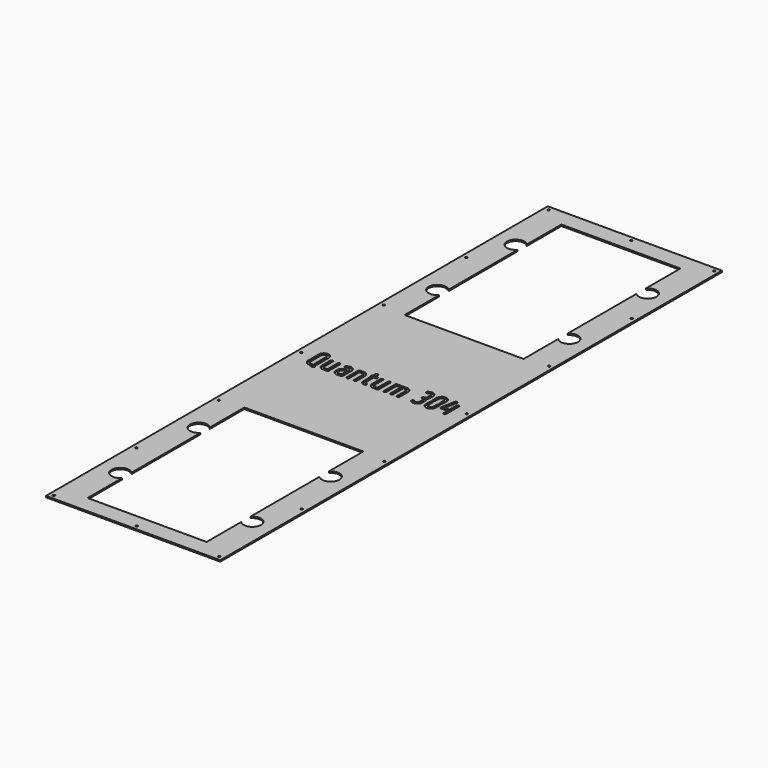
from build123d import *

# Parameters (mm, degrees)
F0_W     = 254
F0_H     = 914.4
F0_R     = 1.5750032
F1_DEPTH = 2.032


# Not quite as in the source:
# - ends of sketch curves that miss each other by under 0.0002 mm in the source are joined


with BuildPart() as f1:
    # F0 (on Top) → F1 (new body)
    with BuildSketch(Plane.XY):
        Rectangle(F0_W, F0_H)
        with Locations((-120.65, -450.85)):
            Circle(F0_R, mode=Mode.SUBTRACT)
        with Locations((-120.65, -300.5666582)):
            Circle(F0_R, mode=Mode.SUBTRACT)
        with Locations((-120.65, -150.2833418)):
            Circle(F0_R, mode=Mode.SUBTRACT)
        Polygon((-88.2005348, -19.8040498), (-88.2997472, -19.8288656), (-88.4237754, -19.853656), (-88.5229878, -19.8784718), (-88.6222002, -19.8784718), (-88.7214126, -19.8784718), (-88.7958346, -19.8784718), (-88.895047, -19.8784718), (-88.969469, -19.8784718), (-89.043891, -19.853656), (-89.1182876, -19.853656), (-89.1927096, -19.8288656), (-89.2671316, -19.8040498), (-89.366344, -19.7792594), (-97.1302096, -17.1251372), (-97.626297, -16.9515028), (-98.0727782, -16.753078), (-98.5192848, -16.5298374), (-98.9161598, -16.3065968), (-99.3130348, -16.0585404), (-99.685094, -15.810484), (-100.007547, -15.5376372), (-100.3300254, -15.24), (-100.8261128, -14.694281), (-101.272594, -14.1237716), (-101.6198628, -13.5284718), (-101.9423158, -12.9083562), (-102.1655564, -12.238609), (-102.3391908, -11.5688872), (-102.4384032, -10.8495592), (-102.463219, -10.1054154), (-102.463219, 9.2422472), (-102.4384032, 9.9615752), (-102.3391908, 10.6809032), (-102.1655564, 11.350625), (-101.9423158, 12.0203722), (-101.6198628, 12.6404878), (-101.272594, 13.2357876), (-100.8261128, 13.806297), (-100.3300254, 14.352016), (-99.7843064, 14.8481034), (-99.213797, 15.2945846), (-98.6184972, 15.6418534), (-97.9983816, 15.9643064), (-97.3286598, 16.187547), (-96.6589126, 16.3611814), (-95.9395846, 16.4603938), (-95.1954408, 16.4852096), (-94.4761128, 16.4603938), (-93.7567848, 16.3611814), (-93.0870376, 16.187547), (-92.4173158, 15.9643064), (-91.7972002, 15.6418534), (-91.2019004, 15.2945846), (-90.631391, 14.8481034), (-90.085672, 14.352016), (-89.5895846, 13.806297), (-89.1431034, 13.2357876), (-88.7958346, 12.6404878), (-88.4733816, 12.0203722), (-88.250141, 11.350625), (-88.0765066, 10.6809032), (-87.9772688, 9.9615752), (-87.9524784, 9.2422472), (-87.9524784, -10.1054154), (-87.9524784, -10.328656), (-87.9524784, -10.5518966), (-87.9772688, -10.7751372), (-88.0020846, -10.9983778), (-88.0269004, -11.196828), (-88.0516908, -11.4200686), (-88.0765066, -11.6184934), (-88.1261128, -11.841734), (-88.1509032, -11.9657622), (-88.2005348, -12.1146062), (-88.250141, -12.238609), (-88.2997472, -12.3626372), (-88.3741438, -12.461875), (-88.4485658, -12.5858778), (-88.5477782, -12.6851156), (-88.647016, -12.8091184), (-88.7958346, -12.9331466), (-88.969469, -13.0571748), (-89.1182876, -13.1563872), (-89.291922, -13.2308092), (-89.4655564, -13.3052312), (-89.6391908, -13.3548374), (-89.837641, -13.3796278), (-90.0360658, -13.3796278), (-90.234516, -13.3796278), (-90.4081504, -13.3548374), (-90.6065752, -13.3052312), (-90.7802096, -13.2308092), (-90.9290282, -13.1563872), (-91.1026626, -13.0571748), (-91.2515066, -12.9579624), (-91.4003252, -12.8091184), (-91.5243534, -12.6602998), (-91.6483816, -12.5114812), (-91.747594, -12.3626372), (-91.822016, -12.1890028), (-91.8964126, -12.0153684), (-91.9212284, -11.841734), (-91.9460188, -11.6433092), (-91.9708346, -11.444859), (-91.9708346, -11.3952528), (-91.9708346, -11.3456466), (-91.9708346, -11.2960404), (-91.9708346, -11.2464342), (-91.9460188, -11.196828), (-91.9460188, -11.122406), (-91.9460188, -11.0727998), (-91.9460188, -11.0231936), (-91.9212284, -10.8991654), (-91.8964126, -10.799953), (-91.8716222, -10.6759248), (-91.8468064, -10.5767124), (-91.8468064, -10.4526842), (-91.822016, -10.3534718), (-91.822016, -10.2294436), (-91.822016, -10.1054154), (-91.822016, 9.2422472), (-91.8468064, 9.5647002), (-91.8716222, 9.911969), (-91.9708346, 10.234422), (-92.070047, 10.5320846), (-92.218891, 10.8297472), (-92.3677096, 11.102594), (-92.5909502, 11.3754408), (-92.8141908, 11.6234972), (-93.0622472, 11.8467378), (-93.335094, 12.0699784), (-93.6079408, 12.218797), (-93.9056034, 12.367641), (-94.203266, 12.4668534), (-94.525719, 12.5660658), (-94.8729878, 12.5908816), (-95.1954408, 12.615672), (-95.5427096, 12.5908816), (-95.8899784, 12.5660658), (-96.2124314, 12.4668534), (-96.510094, 12.367641), (-96.8077566, 12.218797), (-97.0806034, 12.0699784), (-97.3534502, 11.8467378), (-97.6015066, 11.6234972), (-97.8247472, 11.3754408), (-98.0479878, 11.102594), (-98.1968064, 10.8297472), (-98.3456504, 10.5320846), (-98.4448628, 10.234422), (-98.5440752, 9.911969), (-98.568891, 9.5647002), (-98.5936814, 9.2422472), (-98.5936814, -10.1054154), (-98.568891, -10.4526842), (-98.5440752, -10.7751372), (-98.4696532, -11.0727998), (-98.3704408, -11.3704624), (-98.2216222, -11.6433092), (-98.0727782, -11.8913656), (-97.8743534, -12.1393966), (-97.6511128, -12.3626372), (-97.4278722, -12.5610874), (-97.1798158, -12.7595122), (-96.9317848, -12.9331466), (-96.6589126, -13.0819906), (-96.4108816, -13.2059934), (-96.113219, -13.3300216), (-95.8403722, -13.429234), (-95.5427096, -13.5284718), (-88.1261128, -16.1081466), (-87.9276626, -16.1825686), (-87.7540282, -16.281781), (-87.6052096, -16.3809934), (-87.456391, -16.5050216), (-87.307547, -16.6290498), (-87.1835188, -16.7778684), (-87.0843064, -16.9267124), (-86.985094, -17.1003468), (-86.9354878, -17.224375), (-86.910672, -17.3235874), (-86.8610658, -17.4227998), (-86.8362754, -17.546828), (-86.8114596, -17.6460404), (-86.8114596, -17.7452528), (-86.7866438, -17.8444906), (-86.7866438, -17.943703), (-86.7866438, -18.018125), (-86.7866438, -18.0925216), (-86.8114596, -18.1669436), (-86.8114596, -18.2413656), (-86.8362754, -18.3157622), (-86.8362754, -18.3901842), (-86.8610658, -18.4893966), (-86.8858816, -18.5638186), (-86.9602782, -18.737453), (-87.059516, -18.9110874), (-87.1587284, -19.0847218), (-87.2579408, -19.2335404), (-87.4067848, -19.3575686), (-87.5556034, -19.4815968), (-87.704422, -19.605625), (-87.8780564, -19.7048374), (-87.9772688, -19.7296278), (-88.101297, -19.7792594), align=None, mode=Mode.SUBTRACT)
        Polygon((-82.4954408, -11.0727998), (-82.5946532, -10.3782622), (-82.6442848, -9.6341184), (-82.6442848, 5.3727096), (-82.619469, 5.546344), (-82.5946532, 5.7447688), (-82.545047, 5.9184032), (-82.4954408, 6.0920376), (-82.4210188, 6.265672), (-82.3218064, 6.4393064), (-82.1977782, 6.588125), (-82.0737754, 6.736969), (-81.9249314, 6.8609972), (-81.7761128, 6.985), (-81.6024784, 7.0842378), (-81.428844, 7.1586344), (-81.2552096, 7.208266), (-81.0815752, 7.2578722), (-80.8831504, 7.2826626), (-80.709516, 7.3074784), (-80.5110658, 7.2826626), (-80.312641, 7.2578722), (-80.1390066, 7.208266), (-79.9653722, 7.1586344), (-79.7917378, 7.0842378), (-79.6181034, 6.985), (-79.4692848, 6.8609972), (-79.3204408, 6.736969), (-79.1964126, 6.588125), (-79.0724098, 6.4393064), (-78.973172, 6.265672), (-78.8987754, 6.0920376), (-78.8491438, 5.9184032), (-78.7995376, 5.7447688), (-78.7747472, 5.546344), (-78.7747472, 5.3727096), (-78.7747472, -9.6341184), (-78.7499314, -9.9813872), (-78.7003252, -10.3038656), (-78.6259032, -10.6263186), (-78.5266908, -10.9239812), (-78.3778722, -11.2216184), (-78.2042378, -11.4944906), (-78.0057876, -11.7673374), (-77.782547, -12.0401842), (-77.5097002, -12.2634248), (-77.2368534, -12.461875), (-76.9640066, -12.635484), (-76.666344, -12.784328), (-76.3686814, -12.8835404), (-76.0462284, -12.9579624), (-75.7237754, -13.0075686), (-75.3765066, -13.032359), (-71.978266, -13.032359), (-71.978266, 5.3727096), (-71.978266, 5.546344), (-71.9534502, 5.7447688), (-71.903844, 5.9184032), (-71.8542378, 6.0920376), (-71.7798158, 6.265672), (-71.6806034, 6.4393064), (-71.5565752, 6.588125), (-71.432547, 6.736969), (-71.2837284, 6.8609972), (-71.1349098, 6.985), (-70.9612754, 7.0842378), (-70.787641, 7.1586344), (-70.6140066, 7.208266), (-70.4403722, 7.2578722), (-70.241922, 7.2826626), (-70.0434972, 7.3074784), (-69.8698628, 7.2826626), (-69.6714126, 7.2578722), (-69.4977782, 7.208266), (-69.3241438, 7.1586344), (-69.1505348, 7.0842378), (-68.9769004, 6.985), (-68.8280564, 6.8609972), (-68.6792378, 6.736969), (-68.5552096, 6.588125), (-68.4311814, 6.4393064), (-68.331969, 6.265672), (-68.257547, 6.0920376), (-68.2079408, 5.9184032), (-68.1583346, 5.7447688), (-68.1335188, 5.546344), (-68.1087284, 5.3727096), (-68.1087284, -14.9671278), (-68.1335188, -15.1407622), (-68.1583346, -15.3392124), (-68.2079408, -15.5128468), (-68.257547, -15.6864812), (-68.331969, -15.8601156), (-68.4311814, -16.03375), (-68.5552096, -16.1825686), (-68.6792378, -16.3313872), (-68.8280564, -16.4554154), (-68.9769004, -16.5794436), (-69.1505348, -16.678656), (-69.3241438, -16.753078), (-69.4977782, -16.8026842), (-69.6714126, -16.8522904), (-69.8698628, -16.8771062), (-70.0434972, -16.9018966), (-75.3765066, -16.9018966), (-76.1206504, -16.8522904), (-76.8151626, -16.753078), (-77.5097002, -16.5794436), (-78.1546316, -16.356203), (-78.7747472, -16.0585404), (-79.3948628, -15.6864812), (-79.9653722, -15.2647904), (-80.5110658, -14.768703), (-81.0071532, -14.222984), (-81.428844, -13.6525), (-81.8009032, -13.032359), (-82.0985658, -12.4122434), (-82.3218064, -11.7673374), align=None, mode=Mode.SUBTRACT)
        Polygon((-62.304422, -7.6745592), (-62.2796316, -6.9304154), (-62.1803938, -6.2358778), (-62.0067848, -5.5413656), (-61.7835188, -4.8964342), (-61.4610658, -4.2763186), (-61.113797, -3.656203), (-60.6673158, -3.0856936), (-60.1712284, -2.54), (-59.6999314, -2.0934934), (-59.1790282, -1.7214342), (-58.6581504, -1.3741654), (-58.1124314, -1.0765028), (-57.541922, -0.8532622), (-56.9466222, -0.6548374), (-56.3265066, -0.5308092), (-55.706391, -0.4315968), (-55.4583346, -0.4563872), (-55.235094, -0.481203), (-55.0366438, -0.5308092), (-54.838219, -0.5804154), (-54.6397688, -0.6796278), (-54.4661598, -0.7788656), (-54.3173158, -0.878078), (-54.1684972, -1.0268966), (-54.044469, -1.1757406), (-53.9204408, -1.3245592), (-53.8212284, -1.4981936), (-53.7468064, -1.6470122), (-53.6724098, -1.8206466), (-53.6227782, -1.994281), (-53.5979878, -2.1927312), (-53.5979878, -2.3663656), (-53.5979878, -2.5647904), (-53.6227782, -2.7632406), (-53.6724098, -2.936875), (-53.7468064, -3.110484), (-53.8212284, -3.2841184), (-53.9204408, -3.4329624), (-54.0196532, -3.581781), (-54.1436814, -3.730625), (-54.2925254, -3.8546278), (-54.4165282, -3.9538656), (-54.5653722, -4.053078), (-54.7141908, -4.1275), (-54.8630348, -4.2018966), (-55.0118534, -4.2515028), (-55.160672, -4.2763186), (-55.3343064, -4.301109), (-55.631969, -4.3507406), (-55.9296316, -4.4003468), (-56.2024784, -4.4747434), (-56.4753252, -4.5987716), (-56.7233816, -4.7227998), (-56.9714126, -4.8964342), (-57.219469, -5.0700686), (-57.4427096, -5.2933092), (-57.6659502, -5.5413656), (-57.8891908, -5.8142124), (-58.0380348, -6.0870592), (-58.1868534, -6.3847218), (-58.2860658, -6.682359), (-58.3852782, -7.0048374), (-58.410094, -7.3272904), (-58.4349098, -7.6745592), (-58.4349098, -9.6341184), (-58.410094, -9.9813872), (-58.3852782, -10.3038656), (-58.2860658, -10.6263186), (-58.1868534, -10.9239812), (-58.0380348, -11.2216184), (-57.8891908, -11.4944906), (-57.6659502, -11.7673374), (-57.4427096, -12.0401842), (-57.1946532, -12.2634248), (-56.9218064, -12.461875), (-56.6489596, -12.635484), (-56.351297, -12.784328), (-56.0536598, -12.8835404), (-55.7311814, -12.9579624), (-55.3839126, -13.0075686), (-55.0366438, -13.032359), (-51.663219, -13.032359), (-51.663219, 0.5109972), (-51.6880348, 0.8334502), (-51.737641, 1.180719), (-51.8120376, 1.503172), (-51.9360658, 1.8008346), (-52.060094, 2.0984972), (-52.2337284, 2.371344), (-52.4321532, 2.6441908), (-52.6553938, 2.8922472), (-52.928266, 3.1154878), (-53.176297, 3.3387284), (-53.4739596, 3.487547), (-53.7468064, 3.636391), (-54.0692848, 3.7356034), (-54.3917378, 3.8348158), (-54.7141908, 3.8596316), (-55.0614596, 3.884422), (-55.4087284, 3.8596316), (-55.7559972, 3.81), (-56.0784502, 3.7356034), (-56.3761128, 3.636391), (-56.6737754, 3.487547), (-56.9714126, 3.3139126), (-57.2442848, 3.1154878), (-57.5171316, 2.8674314), (-57.6411598, 2.7434032), (-57.7899784, 2.619375), (-57.9636128, 2.5201626), (-58.1124314, 2.445766), (-58.2860658, 2.371344), (-58.484516, 2.3217378), (-58.6581504, 2.296922), (-58.881391, 2.296922), (-59.0550254, 2.296922), (-59.2534502, 2.3217378), (-59.4270846, 2.371344), (-59.600719, 2.4209502), (-59.7743534, 2.5201626), (-59.9479878, 2.619375), (-60.0968064, 2.7186128), (-60.2456504, 2.8674314), (-60.3696532, 2.9914596), (-60.4936814, 3.165094), (-60.5928938, 3.3139126), (-60.6673158, 3.487547), (-60.716922, 3.6611814), (-60.7665282, 3.8348158), (-60.791344, 4.033266), (-60.8161598, 4.2316908), (-60.791344, 4.4053252), (-60.7665282, 4.60375), (-60.716922, 4.7773844), (-60.6673158, 4.9510188), (-60.5928938, 5.1246532), (-60.4936814, 5.2734972), (-60.3696532, 5.4223158), (-60.2456504, 5.5711344), (-59.6999314, 6.0920376), (-59.1046316, 6.5385188), (-58.5093064, 6.9106034), (-57.8644004, 7.2330564), (-57.1946532, 7.4811128), (-56.5249314, 7.6299314), (-55.8056034, 7.7539596), (-55.0614596, 7.77875), (-54.3421316, 7.7539596), (-53.6227782, 7.6547472), (-52.9530564, 7.4811128), (-52.2833346, 7.2578722), (-51.663219, 6.9353938), (-51.0678938, 6.588125), (-50.4974098, 6.1416438), (-49.9516908, 5.6455564), (-49.4556034, 5.0998628), (-49.0091222, 4.5293534), (-48.6370376, 3.9340282), (-48.3394004, 3.2891222), (-48.1161598, 2.6441908), (-47.9425254, 1.9496532), (-47.8432876, 1.2303252), (-47.7936814, 0.5109972), (-47.7936814, -14.9671278), (-47.7936814, -15.1407622), (-47.8184972, -15.3392124), (-47.8681034, -15.5128468), (-47.9425254, -15.6864812), (-48.016922, -15.8601156), (-48.1161598, -16.03375), (-48.2401626, -16.1825686), (-48.3641908, -16.3313872), (-48.5130348, -16.4554154), (-48.6618534, -16.5794436), (-48.810672, -16.678656), (-48.9843064, -16.753078), (-49.1579408, -16.8026842), (-49.3315752, -16.8522904), (-49.5300254, -16.8771062), (-49.7284502, -16.9018966), (-55.0366438, -16.9018966), (-55.7807876, -16.8522904), (-56.500141, -16.753078), (-57.1698628, -16.5794436), (-57.8395846, -16.356203), (-58.4597002, -16.0585404), (-59.0550254, -15.6864812), (-59.6255348, -15.2647904), (-60.1712284, -14.768703), (-60.6673158, -14.222984), (-61.113797, -13.6525), (-61.4610658, -13.032359), (-61.7835188, -12.4122434), (-62.0067848, -11.7673374), (-62.1803938, -11.0727998), (-62.2796316, -10.3782622), (-62.304422, -9.6341184), align=None, mode=Mode.SUBTRACT)
        Polygon((-42.3862754, 5.9184032), (-42.3118534, 6.0920376), (-42.2374314, 6.265672), (-42.138219, 6.4393064), (-42.0141908, 6.588125), (-41.8901626, 6.736969), (-41.741344, 6.8609972), (-41.5925254, 6.985), (-41.4436814, 7.0842378), (-41.270047, 7.1586344), (-41.0964126, 7.208266), (-40.9227782, 7.2578722), (-40.7243534, 7.2826626), (-40.5259032, 7.3074784), (-35.2177096, 7.3074784), (-34.4735658, 7.2578722), (-33.7542378, 7.1586344), (-33.084516, 6.985), (-32.4147688, 6.7617594), (-31.7946532, 6.4641222), (-31.1993534, 6.0920376), (-30.628844, 5.6703722), (-30.0831504, 5.1742594), (-29.5870376, 4.6285658), (-29.1405564, 4.0580564), (-28.7932876, 3.4379408), (-28.4708346, 2.8178252), (-28.247594, 2.1728938), (-28.0739596, 1.4783816), (-27.9747472, 0.783844), (-27.9499314, 0.0397002), (-27.9499314, -14.9671278), (-27.9499314, -15.1407622), (-27.9747472, -15.3392124), (-28.0243534, -15.5128468), (-28.0987754, -15.6864812), (-28.173172, -15.8601156), (-28.2724098, -16.03375), (-28.3964126, -16.1825686), (-28.5204408, -16.3313872), (-28.6692848, -16.4554154), (-28.8181034, -16.5794436), (-28.966922, -16.678656), (-29.1405564, -16.753078), (-29.3141908, -16.8026842), (-29.4878252, -16.8522904), (-29.6862754, -16.8771062), (-29.8847002, -16.9018966), (-30.0831504, -16.8771062), (-30.2815752, -16.8522904), (-30.4552096, -16.8026842), (-30.628844, -16.753078), (-30.8024784, -16.678656), (-30.951297, -16.5794436), (-31.100141, -16.4554154), (-31.2489596, -16.3313872), (-31.3729878, -16.1825686), (-31.497016, -16.03375), (-31.5962284, -15.8601156), (-31.6706504, -15.6864812), (-31.745047, -15.5128468), (-31.7946532, -15.3392124), (-31.819469, -15.1407622), (-31.819469, -14.9671278), (-31.819469, 0.0397002), (-31.8442848, 0.386969), (-31.8690752, 0.709422), (-31.9682876, 1.031875), (-32.0675254, 1.3295376), (-32.216344, 1.6272002), (-32.3651626, 1.900047), (-32.5884032, 2.1728938), (-32.8116438, 2.445766), (-33.0597002, 2.6690066), (-33.332547, 2.8674314), (-33.6053938, 3.0410658), (-33.9030564, 3.1898844), (-34.200719, 3.2891222), (-34.523172, 3.3635188), (-34.8704408, 3.413125), (-35.2177096, 3.4379408), (-38.5911598, 3.4379408), (-38.5911598, -14.9671278), (-38.5911598, -15.1407622), (-38.6159502, -15.3392124), (-38.6655564, -15.5128468), (-38.7399784, -15.6864812), (-38.8144004, -15.8601156), (-38.9136128, -16.03375), (-39.037641, -16.1825686), (-39.1616438, -16.3313872), (-39.3104878, -16.4554154), (-39.4593064, -16.5794436), (-39.6081504, -16.678656), (-39.7817848, -16.753078), (-39.9553938, -16.8026842), (-40.1290282, -16.8522904), (-40.3274784, -16.8771062), (-40.5259032, -16.9018966), (-40.7243534, -16.8771062), (-40.9227782, -16.8522904), (-41.0964126, -16.8026842), (-41.270047, -16.753078), (-41.4436814, -16.678656), (-41.5925254, -16.5794436), (-41.741344, -16.4554154), (-41.8901626, -16.3313872), (-42.0141908, -16.1825686), (-42.138219, -16.03375), (-42.2374314, -15.8601156), (-42.3118534, -15.6864812), (-42.3862754, -15.5128468), (-42.4358816, -15.3392124), (-42.460672, -15.1407622), (-42.460672, -14.9671278), (-42.460672, 5.3727096), (-42.460672, 5.546344), (-42.4358816, 5.7447688), align=None, mode=Mode.SUBTRACT)
        Polygon((-22.3440752, 3.81), (-22.4432876, 3.9092378), (-22.5425254, 4.0084502), (-22.691344, 4.1572688), (-22.7905564, 4.3061128), (-22.8897688, 4.4797472), (-22.9890066, 4.6285658), (-23.0386128, 4.8022002), (-23.088219, 4.9758346), (-23.1130348, 5.1742594), (-23.1130348, 5.3727096), (-23.1130348, 5.546344), (-23.088219, 5.7447688), (-23.0386128, 5.9184032), (-22.9890066, 6.0920376), (-22.8897688, 6.265672), (-22.7905564, 6.4393064), (-22.691344, 6.588125), (-22.5425254, 6.736969), (-22.4432876, 6.8361814), (-22.3440752, 6.9106034), (-22.2448628, 6.985), (-22.1208346, 7.059422), (-22.0216222, 7.1090282), (-21.897594, 7.1586344), (-21.7735658, 7.208266), (-21.6495376, 7.2578722), (-21.6495376, 11.1522002), (-21.6495376, 11.3258346), (-21.6247472, 11.5242594), (-21.575141, 11.6978938), (-21.500719, 11.8715282), (-21.426297, 12.0451626), (-21.3270846, 12.218797), (-21.2030564, 12.367641), (-21.0790282, 12.5164596), (-20.9302096, 12.6404878), (-20.7565752, 12.764516), (-20.6077566, 12.8637284), (-20.4341222, 12.938125), (-20.2604878, 12.9877566), (-20.0868534, 13.0373628), (-19.913219, 13.0621532), (-19.7147688, 13.086969), (-19.516344, 13.0621532), (-19.3178938, 13.0373628), (-19.1442848, 12.9877566), (-18.9706504, 12.938125), (-18.797016, 12.8637284), (-18.648172, 12.764516), (-18.4993534, 12.6404878), (-18.3505348, 12.5164596), (-18.2265066, 12.367641), (-18.1024784, 12.218797), (-18.003266, 12.0451626), (-17.928844, 11.8715282), (-17.854422, 11.6978938), (-17.8048158, 11.5242594), (-17.7800254, 11.3258346), (-17.7800254, 11.1522002), (-17.7800254, 7.3074784), (-15.3491438, 7.3074784), (-15.1755348, 7.2826626), (-14.9770846, 7.2578722), (-14.8034502, 7.208266), (-14.6298158, 7.1586344), (-14.4561814, 7.0842378), (-14.282547, 6.985), (-14.1337284, 6.8609972), (-13.9849098, 6.736969), (-13.8608816, 6.588125), (-13.7368534, 6.4393064), (-13.637641, 6.265672), (-13.563219, 6.0920376), (-13.5136128, 5.9184032), (-13.4640066, 5.7447688), (-13.4391908, 5.546344), (-13.4144004, 5.3727096), (-13.4391908, 5.1742594), (-13.4640066, 4.9758346), (-13.5136128, 4.8022002), (-13.563219, 4.6285658), (-13.637641, 4.4549314), (-13.7368534, 4.281297), (-13.8608816, 4.1324784), (-13.9849098, 3.9836344), (-14.1337284, 3.8596316), (-14.282547, 3.7356034), (-14.4561814, 3.636391), (-14.6298158, 3.561969), (-14.8034502, 3.5123628), (-14.9770846, 3.4627566), (-15.1755348, 3.4379408), (-15.3491438, 3.4379408), (-17.7800254, 3.4379408), (-17.7800254, -10.6015028), (-17.7800254, -10.8495592), (-17.7303938, -11.0976156), (-17.6807876, -11.3208562), (-17.606391, -11.5440968), (-17.5071532, -11.7425216), (-17.3831504, -11.9409718), (-17.2343064, -12.1393966), (-17.0854878, -12.313031), (-16.8870376, -12.4866654), (-16.7134032, -12.635484), (-16.5149784, -12.7347218), (-16.2917378, -12.8339342), (-16.0684972, -12.9331466), (-15.8452566, -12.9827528), (-15.622016, -13.0075686), (-15.3491438, -13.032359), (-15.150719, -13.032359), (-14.9770846, -13.0571748), (-14.7786598, -13.106781), (-14.6050254, -13.1563872), (-14.431391, -13.255625), (-14.282547, -13.3548374), (-14.1089126, -13.4540498), (-13.960094, -13.6028684), (-13.8360658, -13.7517124), (-13.7120376, -13.900531), (-13.6128252, -14.0741654), (-13.5384032, -14.222984), (-13.488797, -14.3966184), (-13.4391908, -14.5702528), (-13.4144004, -14.768703), (-13.4144004, -14.9671278), (-13.4144004, -15.1407622), (-13.4391908, -15.3392124), (-13.488797, -15.5128468), (-13.5384032, -15.6864812), (-13.6128252, -15.8601156), (-13.7120376, -16.03375), (-13.8360658, -16.1825686), (-13.960094, -16.3313872), (-14.1089126, -16.4554154), (-14.282547, -16.5794436), (-14.431391, -16.678656), (-14.6050254, -16.753078), (-14.7786598, -16.8026842), (-14.9770846, -16.8522904), (-15.150719, -16.8771062), (-15.3491438, -16.9018966), (-15.9940752, -16.8522904), (-16.6141908, -16.7778684), (-17.209516, -16.6290498), (-17.7552096, -16.430625), (-18.3009032, -16.1577528), (-18.8218064, -15.8601156), (-19.3178938, -15.4632406), (-19.7891908, -15.0415498), (-20.235672, -14.5702528), (-20.6077566, -14.0741654), (-20.9302096, -13.5532622), (-21.178266, -13.0075686), (-21.4015066, -12.4370592), (-21.5255348, -11.841734), (-21.6247472, -11.2464342), (-21.6495376, -10.6015028), (-21.6495376, 3.4627566), (-21.7735658, 3.5123628), (-21.897594, 3.561969), (-22.0216222, 3.6115752), (-22.1208346, 3.6611814), (-22.2448628, 3.7356034), align=None, mode=Mode.SUBTRACT)
        Polygon((-9.4208346, -11.0727998), (-9.520047, -10.3782622), (-9.5696532, -9.6341184), (-9.5696532, 5.3727096), (-9.5448628, 5.546344), (-9.520047, 5.7447688), (-9.4704408, 5.9184032), (-9.4208346, 6.0920376), (-9.3464126, 6.265672), (-9.2472002, 6.4393064), (-9.123172, 6.588125), (-8.9991438, 6.736969), (-8.8503252, 6.8609972), (-8.7015066, 6.985), (-8.5278722, 7.0842378), (-8.3542378, 7.1586344), (-8.1806034, 7.208266), (-8.006969, 7.2578722), (-7.8085188, 7.2826626), (-7.6349098, 7.3074784), (-7.4364596, 7.2826626), (-7.2380348, 7.2578722), (-7.0644004, 7.208266), (-6.890766, 7.1586344), (-6.7171316, 7.0842378), (-6.5434972, 6.985), (-6.3946532, 6.8609972), (-6.2458346, 6.736969), (-6.1218064, 6.588125), (-5.9977782, 6.4393064), (-5.8985658, 6.265672), (-5.8241438, 6.0920376), (-5.7745376, 5.9184032), (-5.7249314, 5.7447688), (-5.700141, 5.546344), (-5.700141, 5.3727096), (-5.700141, -9.6341184), (-5.6753252, -9.9813872), (-5.625719, -10.3038656), (-5.551297, -10.6263186), (-5.4520846, -10.9239812), (-5.303266, -11.2216184), (-5.1296316, -11.4944906), (-4.9311814, -11.7673374), (-4.7079408, -12.0401842), (-4.435094, -12.2634248), (-4.1622472, -12.461875), (-3.8894004, -12.635484), (-3.5917378, -12.784328), (-3.2940752, -12.8835404), (-2.9716222, -12.9579624), (-2.6491438, -13.0075686), (-2.3019004, -13.032359), (1.0963402, -13.032359), (1.0963402, 5.3727096), (1.0963402, 5.546344), (1.121156, 5.7447688), (1.1707622, 5.9184032), (1.2203684, 6.0920376), (1.2947904, 6.265672), (1.3940028, 6.4393064), (1.518031, 6.588125), (1.6420592, 6.736969), (1.7908778, 6.8609972), (1.9397218, 6.985), (2.1133562, 7.0842378), (2.2869652, 7.1586344), (2.4605996, 7.208266), (2.634234, 7.2578722), (2.8326842, 7.2826626), (3.031109, 7.3074784), (3.2047434, 7.2826626), (3.4031936, 7.2578722), (3.576828, 7.208266), (3.7504624, 7.1586344), (3.9240968, 7.0842378), (4.0977312, 6.985), (4.2465498, 6.8609972), (4.3953684, 6.736969), (4.5193966, 6.588125), (4.6434248, 6.4393064), (4.7426372, 6.265672), (4.8170592, 6.0920376), (4.8666654, 5.9184032), (4.9162716, 5.7447688), (4.9410874, 5.546344), (4.9658778, 5.3727096), (4.9658778, -14.9671278), (4.9410874, -15.1407622), (4.9162716, -15.3392124), (4.8666654, -15.5128468), (4.8170592, -15.6864812), (4.7426372, -15.8601156), (4.6434248, -16.03375), (4.5193966, -16.1825686), (4.3953684, -16.3313872), (4.2465498, -16.4554154), (4.0977312, -16.5794436), (3.9240968, -16.678656), (3.7504624, -16.753078), (3.576828, -16.8026842), (3.4031936, -16.8522904), (3.2047434, -16.8771062), (3.031109, -16.9018966), (-2.3019004, -16.9018966), (-3.0460188, -16.8522904), (-3.7405564, -16.753078), (-4.435094, -16.5794436), (-5.0800254, -16.356203), (-5.700141, -16.0585404), (-6.3202566, -15.6864812), (-6.890766, -15.2647904), (-7.4364596, -14.768703), (-7.932547, -14.222984), (-8.3542378, -13.6525), (-8.726297, -13.032359), (-9.0239596, -12.4122434), (-9.2472002, -11.7673374), align=None, mode=Mode.SUBTRACT)
        with Locations((0, -450.85)):
            Circle(F0_R, mode=Mode.SUBTRACT)
        with BuildLine():
            Line((-86.7791, -209.0872374), (-86.7791, -146.05))
            Line((-86.7791, -146.05), (86.7791, -146.05))
            Line((86.7791, -146.05), (86.7791, -209.0872374))
            ThreePointArc((86.7791, -209.0872374), (109.0041, -217.4875), (86.7791010851, -225.887761643))
            Line((86.7791010851, -225.887761643), (86.7791, -351.9622374))
            ThreePointArc((86.7791, -351.9622374), (109.0041, -360.3625), (86.7791010851, -368.762761643))
            Line((86.7791010851, -368.762761643), (86.7791, -431.8))
            Line((86.7791, -431.8), (-86.7791, -431.8))
            Line((-86.7791, -431.8), (-86.7791, -368.7627626))
            ThreePointArc((-86.7791, -368.7627626), (-109.0041, -360.3625), (-86.7791010851, -351.962238357))
            Line((-86.7791010851, -351.962238357), (-86.7791, -225.8877626))
            ThreePointArc((-86.7791, -225.8877626), (-109.0041, -217.4875), (-86.7791, -209.0872374))
        make_face(mode=Mode.SUBTRACT)
        with Locations((120.65, -450.85)):
            Circle(F0_R, mode=Mode.SUBTRACT)
        with Locations((120.65, -300.5666582)):
            Circle(F0_R, mode=Mode.SUBTRACT)
        Polygon((11.8863872, -15.6864812), (11.8119652, -15.5128468), (11.762359, -15.3392124), (11.7375686, -15.1407622), (11.7375686, -14.9671278), (11.7375686, 5.3727096), (11.7375686, 5.546344), (11.762359, 5.7447688), (11.8119652, 5.9184032), (11.8863872, 6.0920376), (11.9608092, 6.265672), (12.0600216, 6.4393064), (12.1840498, 6.588125), (12.308078, 6.736969), (12.4568966, 6.8609972), (12.6057152, 6.985), (12.7545592, 7.0842378), (12.9281936, 7.1586344), (13.101828, 7.208266), (13.2754624, 7.2578722), (13.4738872, 7.2826626), (13.6723374, 7.3074784), (27.711781, 7.3074784), (28.431109, 7.2578722), (29.1504624, 7.1586344), (29.8201842, 6.985), (30.489906, 6.7617594), (31.1100216, 6.4641222), (31.7053468, 6.0920376), (32.2758562, 5.6703722), (32.8215498, 5.1742594), (33.3176372, 4.6285658), (33.7641184, 4.0580564), (34.1113872, 3.4379408), (34.4338402, 2.8178252), (34.6571062, 2.1728938), (34.8307152, 1.4783816), (34.929953, 0.783844), (34.9547434, 0.0397002), (34.9547434, -14.9671278), (34.9547434, -15.1407622), (34.929953, -15.3392124), (34.8803468, -15.5128468), (34.8059248, -15.6864812), (34.7315028, -15.8601156), (34.6322904, -16.03375), (34.5082622, -16.1825686), (34.384234, -16.3313872), (34.2354154, -16.4554154), (34.0865968, -16.5794436), (33.9377528, -16.678656), (33.7641184, -16.753078), (33.590484, -16.8026842), (33.4168496, -16.8522904), (33.2184248, -16.8771062), (33.0199746, -16.9018966), (32.8215498, -16.8771062), (32.6230996, -16.8522904), (32.4494652, -16.8026842), (32.2758562, -16.753078), (32.1022218, -16.678656), (31.9533778, -16.5794436), (31.8045592, -16.4554154), (31.6557152, -16.3313872), (31.5317124, -16.1825686), (31.4076842, -16.03375), (31.3084718, -15.8601156), (31.2340498, -15.6864812), (31.1596278, -15.5128468), (31.1100216, -15.3392124), (31.0852312, -15.1407622), (31.0852312, -14.9671278), (31.0852312, 0.0397002), (31.0604154, 0.386969), (31.0355996, 0.709422), (30.9363872, 1.031875), (30.8371748, 1.3295376), (30.6883562, 1.6272002), (30.5395122, 1.900047), (30.3162716, 2.1728938), (30.093031, 2.445766), (29.8449746, 2.6690066), (29.5721278, 2.8674314), (29.299281, 3.0410658), (29.0016184, 3.1898844), (28.7039812, 3.2891222), (28.3815028, 3.3635188), (28.034234, 3.413125), (27.711781, 3.4379408), (25.2809248, 3.4379408), (25.2809248, -14.9671278), (25.2809248, -15.1407622), (25.256109, -15.3392124), (25.2065028, -15.5128468), (25.1321062, -15.6864812), (25.0576842, -15.8601156), (24.9584718, -16.03375), (24.8344436, -16.1825686), (24.7104154, -16.3313872), (24.5615968, -16.4554154), (24.4127528, -16.5794436), (24.2639342, -16.678656), (24.0902998, -16.753078), (23.9166654, -16.8026842), (23.743031, -16.8522904), (23.5446062, -16.8771062), (23.346156, -16.9018966), (23.1477312, -16.8771062), (22.949281, -16.8522904), (22.7756466, -16.8026842), (22.6020122, -16.753078), (22.4283778, -16.678656), (22.2795592, -16.5794436), (22.1307152, -16.4554154), (21.9818966, -16.3313872), (21.8578684, -16.1825686), (21.7338402, -16.03375), (21.6346278, -15.8601156), (21.5602312, -15.6864812), (21.4858092, -15.5128468), (21.436203, -15.3392124), (21.4113872, -15.1407622), (21.4113872, -14.9671278), (21.4113872, 3.4379408), (15.6071062, 3.4379408), (15.6071062, -14.9671278), (15.6071062, -15.1407622), (15.5822904, -15.3392124), (15.5326842, -15.5128468), (15.4582622, -15.6864812), (15.3838402, -15.8601156), (15.2846278, -16.03375), (15.1605996, -16.1825686), (15.0365968, -16.3313872), (14.8877528, -16.4554154), (14.7389342, -16.5794436), (14.5900902, -16.678656), (14.4164812, -16.753078), (14.2428468, -16.8026842), (14.0692124, -16.8522904), (13.8707622, -16.8771062), (13.6723374, -16.9018966), (13.4738872, -16.8771062), (13.2754624, -16.8522904), (13.101828, -16.8026842), (12.9281936, -16.753078), (12.7545592, -16.678656), (12.6057152, -16.5794436), (12.4568966, -16.4554154), (12.308078, -16.3313872), (12.1840498, -16.1825686), (12.0600216, -16.03375), (11.9608092, -15.8601156), align=None, mode=Mode.SUBTRACT)
        Polygon((51.052984, -14.3470122), (51.0033778, -14.1733778), (50.9785874, -13.974953), (50.9537716, -13.8013186), (50.9785874, -13.6028684), (51.0033778, -13.4044436), (51.052984, -13.2308092), (51.1025902, -13.0571748), (51.1770122, -12.8835404), (51.2762246, -12.7347218), (51.4002528, -12.5610874), (51.524281, -12.4370592), (51.6730996, -12.2882406), (51.8219436, -12.1890028), (51.995578, -12.0897904), (52.1692124, -11.990578), (52.3428468, -11.9409718), (52.5164812, -11.8913656), (52.714906, -11.8665498), (52.8885404, -11.8665498), (53.0869652, -11.8665498), (53.2854154, -11.8913656), (53.4590498, -11.9409718), (53.6326842, -11.990578), (53.8063186, -12.065), (53.979953, -12.1642124), (54.1287716, -12.2882406), (54.2775902, -12.4122434), (54.5504624, -12.6602998), (54.8233092, -12.8835404), (55.1209718, -13.0571748), (55.418609, -13.2059934), (55.7410874, -13.3300216), (56.0635404, -13.4044436), (56.4108092, -13.4540498), (56.7332622, -13.4788656), (57.1053468, -13.4540498), (57.4277998, -13.429234), (57.7502528, -13.3300216), (58.0479154, -13.2308092), (58.345578, -13.0819906), (58.6432152, -12.9331466), (58.8912716, -12.709906), (59.139328, -12.4866654), (59.387359, -12.238609), (59.5858092, -11.9657622), (59.7594436, -11.6929154), (59.8834718, -11.3952528), (59.9826842, -11.0976156), (60.0818966, -10.7751372), (60.1067124, -10.4526842), (60.1315028, -10.1054154), (60.1315028, -4.772406), (60.1315028, -4.524375), (60.0818966, -4.2763186), (60.0322904, -4.053078), (59.9578684, -3.8298374), (59.858656, -3.6313872), (59.7346278, -3.4329624), (59.6105996, -3.2345122), (59.4369652, -3.0608778), (59.2633562, -2.8872434), (59.064906, -2.7384248), (58.8664812, -2.6392124), (58.668031, -2.54), (58.4447904, -2.465578), (58.2215498, -2.391156), (57.9734934, -2.3663656), (57.7254624, -2.3663656), (57.7006466, -2.3663656), (57.5270122, -2.3415498), (57.3285874, -2.316734), (57.154953, -2.2671278), (56.9813186, -2.2175216), (56.8076842, -2.1183092), (56.6340498, -2.0190968), (56.4852312, -1.919859), (56.3363872, -1.7710404), (56.212359, -1.6222218), (56.0883562, -1.4733778), (55.9891184, -1.2997434), (55.9147218, -1.1509248), (55.8650902, -0.9772904), (55.815484, -0.803656), (55.7906936, -0.6052312), (55.7658778, -0.4315968), (55.7906936, -0.2331466), (55.815484, -0.0347218), (55.8650902, 0.1389126), (55.9147218, 0.312547), (55.9891184, 0.4861814), (56.0883562, 0.6598158), (56.212359, 0.8086344), (56.3363872, 0.9574784), (56.4852312, 1.0815066), (56.6340498, 1.2055094), (56.8076842, 1.3047472), (56.9813186, 1.3791438), (57.154953, 1.42875), (57.3285874, 1.4783816), (57.5270122, 1.503172), (57.7006466, 1.503172), (57.7254624, 1.503172), (57.9734934, 1.5279878), (58.2215498, 1.5527782), (58.4447904, 1.6023844), (58.668031, 1.7016222), (58.8664812, 1.8008346), (59.064906, 1.900047), (59.2633562, 2.048891), (59.4369652, 2.2225), (59.6105996, 2.3961344), (59.7346278, 2.5945846), (59.858656, 2.7930094), (59.9578684, 2.9914596), (60.0322904, 3.2147002), (60.0818966, 3.4379408), (60.1315028, 3.6859972), (60.1315028, 3.9340282), (60.1315028, 9.2422472), (60.1067124, 9.589516), (60.0818966, 9.911969), (59.9826842, 10.234422), (59.8834718, 10.5320846), (59.7594436, 10.8297472), (59.5858092, 11.102594), (59.387359, 11.3754408), (59.139328, 11.6234972), (58.8912716, 11.8467378), (58.6432152, 12.0699784), (58.345578, 12.218797), (58.0479154, 12.367641), (57.7502528, 12.4668534), (57.4277998, 12.5660658), (57.1053468, 12.5908816), (56.7332622, 12.615672), (56.4108092, 12.5908816), (56.0635404, 12.54125), (55.7410874, 12.4668534), (55.4434248, 12.367641), (55.1457622, 12.218797), (54.8480996, 12.0203722), (54.5504624, 11.821922), (54.2775902, 11.573891), (54.1287716, 11.4498628), (53.979953, 11.3258346), (53.8063186, 11.2266222), (53.6326842, 11.1522002), (53.4590498, 11.0777782), (53.2854154, 11.028172), (53.0869652, 11.0033816), (52.8885404, 11.0033816), (52.714906, 11.0033816), (52.5164812, 11.028172), (52.3428468, 11.0777782), (52.1692124, 11.1273844), (51.995578, 11.2266222), (51.8219436, 11.3258346), (51.6730996, 11.425047), (51.524281, 11.573891), (51.4002528, 11.6978938), (51.2762246, 11.8715282), (51.1770122, 12.0203722), (51.1025902, 12.1940066), (51.052984, 12.367641), (51.0033778, 12.54125), (50.9785874, 12.7397002), (50.9537716, 12.938125), (50.9785874, 13.1117594), (51.0033778, 13.3102096), (51.052984, 13.483844), (51.1025902, 13.6574784), (51.201828, 13.8311128), (51.3010404, 13.9799314), (51.4002528, 14.12875), (51.5490968, 14.277594), (52.1196062, 14.7984972), (52.6900902, 15.2697688), (53.3102312, 15.6418534), (53.9551372, 15.9643064), (54.6000686, 16.187547), (55.2946062, 16.3611814), (56.0139342, 16.4852096), (56.7332622, 16.51), (57.477406, 16.4852096), (58.196734, 16.3859972), (58.8664812, 16.2123628), (59.536203, 15.9891222), (60.1563186, 15.6666438), (60.7516184, 15.319375), (61.3221278, 14.8728938), (61.8678468, 14.3768064), (62.3639342, 13.8311128), (62.8104154, 13.2606034), (63.1576842, 12.6652782), (63.4801372, 12.0451626), (63.7033778, 11.3754408), (63.8770122, 10.705719), (63.9762246, 9.986391), (64.0010404, 9.2422472), (64.0010404, 3.9340282), (63.9762246, 3.2891222), (63.901828, 2.693797), (63.752984, 2.0984972), (63.5545592, 1.5527782), (63.3065028, 1.031875), (63.0088402, 0.5109972), (62.636781, 0.0397002), (62.239906, -0.4315968), (62.636781, -0.878078), (63.0088402, -1.349375), (63.3065028, -1.8702528), (63.5545592, -2.391156), (63.752984, -2.936875), (63.901828, -3.5321748), (63.9762246, -4.1275), (64.0010404, -4.772406), (64.0010404, -10.1054154), (63.9762246, -10.8495592), (63.8770122, -11.5688872), (63.7033778, -12.238609), (63.4801372, -12.9083562), (63.1576842, -13.5284718), (62.8104154, -14.1237716), (62.3639342, -14.694281), (61.8678468, -15.24), (61.3221278, -15.7360874), (60.7516184, -16.1825686), (60.1563186, -16.5298374), (59.536203, -16.8522904), (58.8664812, -17.075531), (58.196734, -17.2491654), (57.477406, -17.3483778), (56.7332622, -17.3731936), (56.0139342, -17.3483778), (55.2946062, -17.224375), (54.6000686, -17.0507406), (53.9551372, -16.8275), (53.3102312, -16.5050216), (52.6900902, -16.1329624), (52.1196062, -15.6616654), (51.5490968, -15.1407622), (51.4002528, -14.9919436), (51.3010404, -14.843125), (51.201828, -14.694281), (51.1025902, -14.5206466), align=None, mode=Mode.SUBTRACT)
        with Locations((120.65, -150.2833418)):
            Circle(F0_R, mode=Mode.SUBTRACT)
        Polygon((73.1787716, -10.4526842), (73.2283778, -10.799953), (73.3027998, -11.122406), (73.4020122, -11.4200686), (73.5508562, -11.7177312), (73.7244652, -11.990578), (73.9229154, -12.2634248), (74.146156, -12.5114812), (74.4190028, -12.7347218), (74.6918496, -12.9579624), (74.9647218, -13.106781), (75.262359, -13.255625), (75.5600216, -13.3548374), (75.8824746, -13.4540498), (76.204953, -13.4788656), (76.5522218, -13.503656), (76.8994652, -13.4788656), (77.2219436, -13.4540498), (77.5443966, -13.3548374), (77.8420592, -13.255625), (78.1397218, -13.106781), (78.4125686, -12.9579624), (78.6854154, -12.7347218), (78.9582622, -12.5114812), (79.1815028, -12.2634248), (79.379953, -11.990578), (79.5535874, -11.7177312), (79.702406, -11.4200686), (79.8016184, -11.122406), (79.8760404, -10.799953), (79.9256466, -10.4526842), (79.9504624, -10.1054154), (79.9504624, -3.3585404), (79.9504624, -3.184906), (79.9752528, -2.9864812), (80.024859, -2.8128468), (80.0744652, -2.6392124), (80.1488872, -2.465578), (80.2480996, -2.2919436), (80.3721278, -2.143125), (80.496156, -1.994281), (80.6449746, -1.8702528), (80.7938186, -1.74625), (80.967453, -1.6470122), (81.1410874, -1.5726156), (81.3147218, -1.522984), (81.4883562, -1.4733778), (81.686781, -1.4485874), (81.8852312, -1.4237716), (82.0588402, -1.4485874), (82.2572904, -1.4733778), (82.4309248, -1.522984), (82.6045592, -1.5726156), (82.7781936, -1.6470122), (82.951828, -1.74625), (83.1006466, -1.8702528), (83.2494652, -1.994281), (83.3734934, -2.143125), (83.4975216, -2.2919436), (83.596734, -2.465578), (83.671156, -2.6392124), (83.7207622, -2.8128468), (83.7703684, -2.9864812), (83.7951842, -3.184906), (83.8199746, -3.3585404), (83.8199746, -10.1054154), (83.7703684, -10.8495592), (83.671156, -11.5688872), (83.4975216, -12.238609), (83.274281, -12.9083562), (82.9766184, -13.5284718), (82.6045592, -14.1237716), (82.1828684, -14.694281), (81.686781, -15.24), (81.1410874, -15.7360874), (80.570578, -16.1825686), (79.9504624, -16.5298374), (79.3303468, -16.8522904), (78.6854154, -17.075531), (77.9908778, -17.2491654), (77.2963402, -17.3483778), (76.5522218, -17.3731936), (75.808078, -17.3483778), (75.1135404, -17.2491654), (74.4190028, -17.075531), (73.7740968, -16.8522904), (73.1539812, -16.5298374), (72.5338402, -16.1825686), (71.9633562, -15.7360874), (71.4176372, -15.24), (70.9215498, -14.694281), (70.499859, -14.1237716), (70.1277998, -13.5284718), (69.8301372, -12.9083562), (69.6068966, -12.238609), (69.4332622, -11.5688872), (69.3340498, -10.8495592), (69.2844436, -10.1054154), (69.2844436, -3.3585404), (69.309234, -3.184906), (69.3340498, -2.9864812), (69.383656, -2.8128468), (69.4332622, -2.6392124), (69.5076842, -2.465578), (69.6068966, -2.2919436), (69.7309248, -2.143125), (69.854953, -1.994281), (70.0037716, -1.8702528), (70.1525902, -1.74625), (70.3262246, -1.6470122), (70.499859, -1.5726156), (70.6734934, -1.522984), (70.8471278, -1.4733778), (71.045578, -1.4485874), (71.2192124, -1.4237716), (71.4176372, -1.4485874), (71.6160874, -1.4733778), (71.7897218, -1.522984), (71.9633562, -1.5726156), (72.1369652, -1.6470122), (72.3105996, -1.74625), (72.4594436, -1.8702528), (72.6082622, -1.994281), (72.7322904, -2.143125), (72.8563186, -2.2919436), (72.955531, -2.465578), (73.029953, -2.6392124), (73.0795592, -2.8128468), (73.1291654, -2.9864812), (73.1539812, -3.184906), (73.1539812, -3.3585404), (73.1539812, -10.1054154), align=None, mode=Mode.SUBTRACT)
        Polygon((87.7639342, -6.831203), (87.714328, -6.6575686), (87.6895122, -6.4591184), (87.6895122, -6.2606936), (87.6895122, -6.1862716), (87.6895122, -6.111875), (87.6895122, -6.037453), (87.6895122, -5.963031), (87.714328, -5.888609), (87.7391184, -5.8390028), (87.7391184, -5.7646062), (87.7639342, -5.715), (91.5590498, 14.0791438), (91.5838402, 14.277594), (91.6334718, 14.4760188), (91.683078, 14.6496532), (91.7574746, 14.8232876), (91.8318966, 14.996922), (91.931109, 15.145766), (92.0303468, 15.2945846), (92.1543496, 15.4434032), (92.3031936, 15.5674314), (92.4520122, 15.6914596), (92.6008562, 15.790672), (92.7496748, 15.865094), (92.9233092, 15.9147002), (93.0969436, 15.9643064), (93.2953684, 15.9891222), (93.4938186, 15.9891222), (93.667453, 15.9891222), (93.8658778, 15.9643064), (94.0395122, 15.9147002), (94.2131466, 15.865094), (94.386781, 15.790672), (94.5604154, 15.6914596), (94.709234, 15.5674314), (94.858078, 15.4434032), (94.9821062, 15.2945846), (95.106109, 15.145766), (95.2053468, 14.9721316), (95.2797434, 14.7984972), (95.3293496, 14.6248628), (95.3789812, 14.4512284), (95.4037716, 14.2527782), (95.4285874, 14.0543534), (95.4037716, 14.0047472), (95.4037716, 13.9303252), (95.4037716, 13.8559032), (95.4037716, 13.7815066), (95.4037716, 13.7070846), (95.3789812, 13.6326626), (95.3789812, 13.5830564), (95.3789812, 13.5086344), (91.9559248, -4.3259248), (98.8020122, -4.3259248), (98.8020122, 8.250047), (98.8020122, 8.4236814), (98.826828, 8.6221316), (98.8764342, 8.795766), (98.9508562, 8.969375), (99.0252528, 9.1430094), (99.1244652, 9.3166438), (99.2484934, 9.4654878), (99.3725216, 9.6143064), (99.5213402, 9.7383346), (99.6701842, 9.8623628), (99.8190028, 9.9615752), (99.9926372, 10.0359972), (100.1662716, 10.0856034), (100.339906, 10.1352096), (100.5383562, 10.16), (100.736781, 10.1848158), (100.9352312, 10.16), (101.133656, 10.1352096), (101.3072904, 10.0856034), (101.4809248, 10.0359972), (101.6545592, 9.9615752), (101.8033778, 9.8623628), (101.9522218, 9.7383346), (102.1010404, 9.6143064), (102.2250686, 9.4654878), (102.3490968, 9.3166438), (102.4483092, 9.1430094), (102.5227312, 8.969375), (102.5971278, 8.795766), (102.646734, 8.6221316), (102.6715498, 8.4236814), (102.6715498, 8.250047), (102.6715498, -14.9671278), (102.6715498, -15.165578), (102.646734, -15.3640028), (102.5971278, -15.5376372), (102.5227312, -15.7112716), (102.4483092, -15.884906), (102.3490968, -16.0585404), (102.2250686, -16.207359), (102.1010404, -16.356203), (101.9522218, -16.4802312), (101.8033778, -16.6042594), (101.6545592, -16.7034718), (101.4809248, -16.7778684), (101.3072904, -16.8275), (101.133656, -16.8771062), (100.9352312, -16.9018966), (100.736781, -16.9018966), (100.5383562, -16.9018966), (100.339906, -16.8771062), (100.1662716, -16.8275), (99.9926372, -16.7778684), (99.8190028, -16.7034718), (99.6701842, -16.6042594), (99.5213402, -16.4802312), (99.3725216, -16.356203), (99.2484934, -16.207359), (99.1244652, -16.0585404), (99.0252528, -15.884906), (98.9508562, -15.7112716), (98.8764342, -15.5376372), (98.826828, -15.3640028), (98.8020122, -15.165578), (98.8020122, -14.9671278), (98.8020122, -8.1954624), (89.624281, -8.1954624), (89.4258562, -8.1954624), (89.227406, -8.1706466), (89.0537716, -8.1210404), (88.8801372, -8.0714342), (88.7065028, -7.9722218), (88.5328684, -7.872984), (88.3840498, -7.7737716), (88.2352312, -7.624953), (88.111203, -7.476109), (87.9871748, -7.3272904), (87.8879624, -7.153656), (87.8135404, -7.0048374), align=None, mode=Mode.SUBTRACT)
        with Locations((-120.65, 0)):
            Circle(F0_R, mode=Mode.SUBTRACT)
        with Locations((-120.65, 150.2833418)):
            Circle(F0_R, mode=Mode.SUBTRACT)
        with Locations((-120.65, 300.5666582)):
            Circle(F0_R, mode=Mode.SUBTRACT)
        with Locations((-120.65, 450.85)):
            Circle(F0_R, mode=Mode.SUBTRACT)
        Polygon((69.2844436, 9.2422472), (69.3340498, 9.986391), (69.4332622, 10.705719), (69.6068966, 11.3754408), (69.8301372, 12.0451626), (70.1277998, 12.6652782), (70.499859, 13.2606034), (70.9215498, 13.8311128), (71.4176372, 14.3768064), (71.9633562, 14.8728938), (72.5338402, 15.319375), (73.1539812, 15.6666438), (73.7740968, 15.9891222), (74.4190028, 16.2123628), (75.1135404, 16.3859972), (75.808078, 16.4852096), (76.5522218, 16.51), (77.2963402, 16.4852096), (77.9908778, 16.3859972), (78.6854154, 16.2123628), (79.3303468, 15.9891222), (79.9504624, 15.6666438), (80.570578, 15.319375), (81.1410874, 14.8728938), (81.686781, 14.3768064), (82.1828684, 13.8311128), (82.6045592, 13.2606034), (82.9766184, 12.6652782), (83.274281, 12.0451626), (83.4975216, 11.3754408), (83.671156, 10.705719), (83.7703684, 9.986391), (83.8199746, 9.2422472), (83.8199746, 2.4953722), (83.7951842, 2.3217378), (83.7703684, 2.1232876), (83.7207622, 1.9496532), (83.671156, 1.7760188), (83.596734, 1.6023844), (83.4975216, 1.42875), (83.3734934, 1.2799314), (83.2494652, 1.1311128), (83.1006466, 1.0070846), (82.951828, 0.8830564), (82.7781936, 0.783844), (82.6045592, 0.709422), (82.4309248, 0.6598158), (82.2572904, 0.6102096), (82.0588402, 0.5853938), (81.8852312, 0.5606034), (81.686781, 0.5853938), (81.4883562, 0.6102096), (81.3147218, 0.6598158), (81.1410874, 0.709422), (80.967453, 0.783844), (80.7938186, 0.8830564), (80.6449746, 1.0070846), (80.496156, 1.1311128), (80.3721278, 1.2799314), (80.2480996, 1.42875), (80.1488872, 1.6023844), (80.0744652, 1.7760188), (80.024859, 1.9496532), (79.9752528, 2.1232876), (79.9504624, 2.3217378), (79.9504624, 2.4953722), (79.9504624, 9.2422472), (79.9256466, 9.589516), (79.8760404, 9.9367594), (79.8016184, 10.2592378), (79.702406, 10.556875), (79.5535874, 10.8545376), (79.379953, 11.1273844), (79.1815028, 11.4002566), (78.9582622, 11.6482876), (78.6854154, 11.8715282), (78.4125686, 12.0699784), (78.1397218, 12.2436128), (77.8420592, 12.3924314), (77.5443966, 12.4916438), (77.2219436, 12.5660658), (76.8994652, 12.615672), (76.5522218, 12.6404878), (76.204953, 12.615672), (75.8824746, 12.5660658), (75.5600216, 12.4916438), (75.262359, 12.3924314), (74.9647218, 12.2436128), (74.6918496, 12.0699784), (74.4190028, 11.8715282), (74.146156, 11.6482876), (73.9229154, 11.4002566), (73.7244652, 11.1273844), (73.5508562, 10.8545376), (73.4020122, 10.556875), (73.3027998, 10.2592378), (73.2283778, 9.9367594), (73.1787716, 9.589516), (73.1539812, 9.2422472), (73.1539812, 2.4953722), (73.1539812, 2.3217378), (73.1291654, 2.1232876), (73.0795592, 1.9496532), (73.029953, 1.7760188), (72.955531, 1.6023844), (72.8563186, 1.42875), (72.7322904, 1.2799314), (72.6082622, 1.1311128), (72.4594436, 1.0070846), (72.3105996, 0.8830564), (72.1369652, 0.783844), (71.9633562, 0.709422), (71.7897218, 0.6598158), (71.6160874, 0.6102096), (71.4176372, 0.5853938), (71.2192124, 0.5606034), (71.045578, 0.5853938), (70.8471278, 0.6102096), (70.6734934, 0.6598158), (70.499859, 0.709422), (70.3262246, 0.783844), (70.1525902, 0.8830564), (70.0037716, 1.0070846), (69.854953, 1.1311128), (69.7309248, 1.2799314), (69.6068966, 1.42875), (69.5076842, 1.6023844), (69.4332622, 1.7760188), (69.383656, 1.9496532), (69.3340498, 2.1232876), (69.309234, 2.3217378), (69.2844436, 2.4953722), align=None, mode=Mode.SUBTRACT)
        with Locations((120.65, 0)):
            Circle(F0_R, mode=Mode.SUBTRACT)
        with Locations((120.65, 150.2833418)):
            Circle(F0_R, mode=Mode.SUBTRACT)
        with BuildLine():
            Line((-86.7791, 368.7627626), (-86.7791, 431.8))
            Line((-86.7791, 431.8), (86.7791, 431.8))
            Line((86.7791, 431.8), (86.7791, 368.7627626))
            ThreePointArc((86.7791, 368.7627626), (109.0041, 360.3625), (86.7791010851, 351.962238357))
            Line((86.7791010851, 351.962238357), (86.7791, 225.8877626))
            ThreePointArc((86.7791, 225.8877626), (109.0041, 217.4875), (86.7791010851, 209.087238357))
            Line((86.7791010851, 209.087238357), (86.7791, 146.05))
            Line((86.7791, 146.05), (-86.7791, 146.05))
            Line((-86.7791, 146.05), (-86.7791, 209.0872374))
            ThreePointArc((-86.7791, 209.0872374), (-109.0041, 217.4875), (-86.7791010851, 225.887761643))
            Line((-86.7791010851, 225.887761643), (-86.7791, 351.9622374))
            ThreePointArc((-86.7791, 351.9622374), (-109.0041, 360.3625), (-86.7791, 368.7627626))
        make_face(mode=Mode.SUBTRACT)
        with Locations((0, 450.85)):
            Circle(F0_R, mode=Mode.SUBTRACT)
        with Locations((120.65, 300.5666582)):
            Circle(F0_R, mode=Mode.SUBTRACT)
        with Locations((120.65, 450.85)):
            Circle(F0_R, mode=Mode.SUBTRACT)
    extrude(amount=F1_DEPTH)


solid = f1.part
